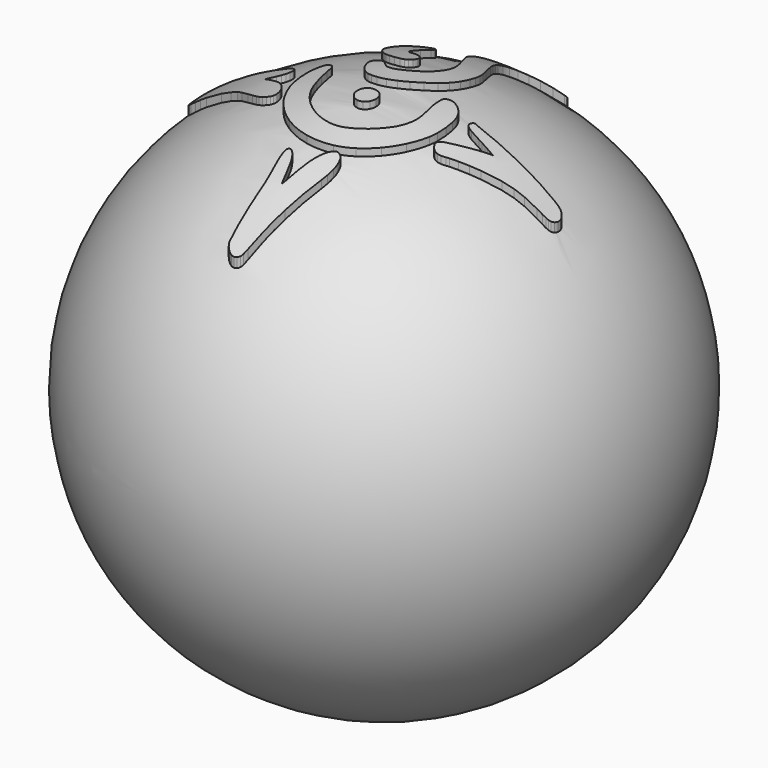
from build123d import *

# Parameters (mm, degrees)
F2_SCALE  = 33.3
F4_DEPTH  = 350
F5_SCALE  = 0.03
F8_SCALE  = 1.4
F9_R      = 2
F10_DEPTH = 25


# Not quite as in the source:
# - ends of sketch curves that miss each other by under 0.0002 mm in the source are joined


with BuildPart() as f1:
    # F0 (on Top) → F1 (revolve)
    with BuildSketch(Plane.XY):
        with BuildLine():
            ThreePointArc((0, 10), (-10, 0), (0, -10))
            Line((0, -10), (0, 10))
        make_face()
    revolve(axis=Axis((0, 0, 0), (0, 1, 0)))


with BuildPart() as f1_1:
    # F2: moved
    add(f1.part.scale(F2_SCALE))

    # F3 (on Top) → F4 (join)
    with BuildSketch(Plane.XY):
        with BuildLine():
            ThreePointArc((33.5839702777, 236.8920416086), (31.2872507857, 235.2369513176), (29.0148242928, 233.5486616119))
            ThreePointArc((29.0148242928, 233.5486616119), (19.1324774159, 225.5301798366), (9.8423522984, 216.8324557031))
            ThreePointArc((9.8423522984, 216.8324557031), (3.1177638553, 209.1003358187), (-2.5120081676, 200.5381260948))
            ThreePointArc((-2.5120081676, 200.5381260948), (-6.4438012248, 192.1284567153), (-9.0353042057, 183.2141060429))
            ThreePointArc((-9.0353042057, 183.2141060429), (-10.4367358481, 173.4113964374), (-10.5813057929, 163.510071961))
            ThreePointArc((-10.5813057929, 163.510071961), (-10.1042819519, 157.7480415442), (-9.2425675321, 152.0308749015))
            ThreePointArc((-9.2425675321, 152.0308749015), (-8.0683662262, 147.037659018), (-6.4222668913, 142.1795410427))
            ThreePointArc((-6.4222668913, 142.1795410427), (-3.8341311453, 136.1498141232), (-0.8786748343, 130.2913730901))
            ThreePointArc((-0.8786748343, 130.2913730901), (4.6685538921, 120.2474903682), (10.345759186, 110.2764991075))
            ThreePointArc((10.345759186, 110.2764991075), (14.4968308965, 102.4949690889), (18.1089318686, 94.4490799463))
            ThreePointArc((18.1089318686, 94.4490799463), (20.3325947861, 87.7758088217), (21.6547046101, 80.8671729519))
            ThreePointArc((21.6547046101, 80.8671729519), (21.933442257, 74.6170651853), (21.2348180753, 68.3998739855))
            ThreePointArc((21.2348180753, 68.3998739855), (19.5614167399, 62.0700272125), (17.0413966753, 56.0271196625))
            ThreePointArc((17.0413966753, 56.0271196625), (14.2722480259, 51.3438477785), (10.8718007094, 47.0967102684))
            ThreePointArc((10.8718007094, 47.0967102684), (6.4493698335, 42.7450902566), (1.6320588081, 38.835102261))
            ThreePointArc((1.6320588081, 38.835102261), (-3.2693678081, 35.5880451103), (-8.4647199209, 32.8356498312))
            ThreePointArc((-8.4647199209, 32.8356498312), (-12.6861471562, 31.3957563266), (-17.119585, 30.9075252801))
            ThreePointArc((-17.119585, 30.9075252801), (-18.5749981899, 30.9588179082), (-20.0231380929, 31.1129263476))
            ThreePointArc((-20.0231380929, 31.1129263476), (-21.0800039659, 31.3548811444), (-22.081829036, 31.7694339301))
            ThreePointArc((-22.081829036, 31.7694339301), (-23.2085403851, 32.4340347627), (-24.2524288095, 33.2223682244))
            ThreePointArc((-24.2524288095, 33.2223682244), (-26.1201182917, 34.8396411796), (-27.9553924433, 36.4936075178))
            ThreePointArc((-27.9553924433, 36.4936075178), (-29.6511377796, 38.0243808047), (-31.3744037529, 39.5241052892))
            ThreePointArc((-31.3744037529, 39.5241052892), (-32.3603682601, 40.2870956891), (-33.4155611268, 40.9510597751))
            ThreePointArc((-33.4155611268, 40.9510597751), (-34.1958978055, 41.3006066899), (-35.0270239713, 41.5014491964))
            ThreePointArc((-35.0270239713, 41.5014491964), (-35.8658550267, 41.5417572719), (-36.6967041013, 41.4194784081))
            ThreePointArc((-36.6967041013, 41.4194784081), (-37.9964275162, 40.9976995728), (-39.2238602532, 40.3972104365))
            ThreePointArc((-39.2238602532, 40.3972104365), (-40.4233299971, 39.6010223307), (-41.5180846961, 38.6660596848))
            ThreePointArc((-41.5180846961, 38.6660596848), (-42.4537917331, 37.6433007258), (-43.2545310552, 36.5117530341))
            ThreePointArc((-43.2545310552, 36.5117530341), (-43.7991045433, 35.4185857778), (-44.1365958304, 34.2448419676))
            ThreePointArc((-44.1365958304, 34.2448419676), (-44.3311387679, 31.90950028), (-44.0309948562, 29.5853700343))
            ThreePointArc((-44.0309948562, 29.5853700343), (-43.1598026618, 26.5326639584), (-42.0249300746, 23.5678614015))
            ThreePointArc((-42.0249300746, 23.5678614015), (-40.4982189899, 20.4151830954), (-38.7147278348, 17.4003221072))
            ThreePointArc((-38.7147278348, 17.4003221072), (-36.7627376663, 14.6873048367), (-34.5602718697, 12.1733691257))
            ThreePointArc((-34.5602718697, 12.1733691257), (-32.4972285983, 10.2580065105), (-30.2358389338, 8.5814391004))
            ThreePointArc((-30.2358389338, 8.5814391004), (-27.9386033944, 7.2780681906), (-25.4883721848, 6.2919474347))
            ThreePointArc((-25.4883721848, 6.2919474347), (-22.7235404396, 5.5680825845), (-19.8920639941, 5.179475077))
            ThreePointArc((-19.8920639941, 5.179475077), (-16.4407701729, 5.0330128077), (-12.9875269897, 5.1224098294))
            ThreePointArc((-12.9875269897, 5.1224098294), (-7.7263055039, 5.755509923), (-2.5780300379, 7.0111081229))
            ThreePointArc((-2.5780300379, 7.0111081229), (2.7682669976, 8.9466005626), (7.9024667665, 11.389757435))
            ThreePointArc((7.9024667665, 11.389757435), (13.2958214566, 14.5927578538), (18.3915086938, 18.2508253897))
            ThreePointArc((18.3915086938, 18.2508253897), (23.754147094, 22.7429501279), (28.8251250537, 27.5618979469))
            ThreePointArc((28.8251250537, 27.5618979469), (33.4797468923, 32.7068050735), (37.6624816046, 38.2421735837))
            ThreePointArc((37.6624816046, 38.2421735837), (41.0387740077, 43.7658663194), (43.7964406901, 49.6229821258))
            ThreePointArc((43.7964406901, 49.6229821258), (45.904591086, 55.7482763417), (47.336918584, 62.0658680708))
            ThreePointArc((47.336918584, 62.0658680708), (48.2013923808, 68.9616610524), (48.4567558849, 75.9067360064))
            ThreePointArc((48.4567558849, 75.9067360064), (48.2830243872, 80.8780020701), (47.8342436997, 85.832017083))
            ThreePointArc((47.8342436997, 85.832017083), (47.1370175393, 90.2919899618), (46.1117340455, 94.6881560124))
            ThreePointArc((46.1117340455, 94.6881560124), (44.6916033909, 99.2773499841), (42.963369873, 103.759612946))
            ThreePointArc((42.963369873, 103.759612946), (40.5613501018, 109.1298002215), (37.9608576069, 114.4067357971))
            ThreePointArc((37.9608576069, 114.4067357971), (32.6470866927, 124.7414153072), (27.3662677803, 135.0929713965))
            ThreePointArc((27.3662677803, 135.0929713965), (24.7259502515, 140.4197225176), (22.1922672104, 145.7980126376))
            ThreePointArc((22.1922672104, 145.7980126376), (20.6601677307, 149.3164912102), (19.2672299611, 152.8923469857))
            ThreePointArc((19.2672299611, 152.8923469857), (18.2940235081, 155.868538738), (17.536259209, 158.9067358325))
            ThreePointArc((17.536259209, 158.9067358325), (16.7190998594, 163.8904603666), (16.3642416365, 168.9282510154))
            ThreePointArc((16.3642416365, 168.9282510154), (16.5213414737, 173.607931726), (17.2169992309, 178.2382829515))
            ThreePointArc((17.2169992309, 178.2382829515), (18.4910489703, 183.0168650293), (20.2695342301, 187.6315198968))
            ThreePointArc((20.2695342301, 187.6315198968), (22.8296254351, 192.8726243488), (25.7284907636, 197.9342271459))
            ThreePointArc((25.7284907636, 197.9342271459), (28.9537669376, 203.2502120973), (32.0973782481, 208.6148938572))
            ThreePointArc((32.0973782481, 208.6148938572), (35.3789821615, 214.3978703308), (38.5879989981, 220.221439001))
            ThreePointArc((38.5879989981, 220.221439001), (41.5839102506, 225.7709084772), (44.5535395691, 231.3344862287))
            ThreePointArc((44.5535395691, 231.3344862287), (44.9905118903, 232.4747939041), (45.139103, 233.686886))
            ThreePointArc((45.139103, 233.686886), (45.0470188997, 234.6434926782), (44.774146878, 235.5649679507))
            ThreePointArc((44.774146878, 235.5649679507), (44.3211975486, 236.4606147714), (43.7242942718, 237.267493239))
            ThreePointArc((43.7242942718, 237.267493239), (42.9700203597, 237.9983716709), (42.1090869519, 238.5999579178))
            ThreePointArc((42.1090869519, 238.5999579178), (41.1398732263, 239.0758936063), (40.1113668985, 239.4046255777))
            ThreePointArc((40.1113668985, 239.4046255777), (39.2636176129, 239.5027838805), (38.4169479014, 239.3957113921))
            ThreePointArc((38.4169479014, 239.3957113921), (37.3828331438, 239.0688465307), (36.3951172895, 238.6209054515))
            ThreePointArc((36.3951172895, 238.6209054515), (34.9610957305, 237.8027303056), (33.5839702777, 236.8920416086))
        make_face()
        with BuildLine():
            ThreePointArc((-42.323086763, 129.1738635543), (-44.1393310136, 128.1627035744), (-45.9151157273, 127.0820665709))
            ThreePointArc((-45.9151157273, 127.0820665709), (-50.1260663332, 123.9751883225), (-53.8649160591, 120.3137950525))
            ThreePointArc((-53.8649160591, 120.3137950525), (-57.1547961085, 116.086062654), (-59.8694062449, 111.4678461233))
            ThreePointArc((-59.8694062449, 111.4678461233), (-62.0590099734, 106.3507303256), (-63.5973965422, 101.0016551201))
            ThreePointArc((-63.5973965422, 101.0016551201), (-64.540269546, 95.2728172325), (-64.8511271886, 89.475235001))
            ThreePointArc((-64.8511271886, 89.475235001), (-64.7217148896, 86.1283645355), (-64.3423022831, 82.800552109))
            ThreePointArc((-64.3423022831, 82.800552109), (-63.7415741406, 79.9469143788), (-62.8227642257, 77.1792599106))
            ThreePointArc((-62.8227642257, 77.1792599106), (-61.6381479464, 74.6412940159), (-60.1599131773, 72.2623428746))
            ThreePointArc((-60.1599131773, 72.2623428746), (-58.3046440662, 69.8898008927), (-56.2304288842, 67.7060861211))
            ThreePointArc((-56.2304288842, 67.7060861211), (-54.0105104417, 65.773116141), (-51.6200521128, 64.0555248264))
            ThreePointArc((-51.6200521128, 64.0555248264), (-49.1742690519, 62.6436953185), (-46.5932000138, 61.4977459638))
            ThreePointArc((-46.5932000138, 61.4977459638), (-43.7334124454, 60.5616789062), (-40.7961929219, 59.9079604538))
            ThreePointArc((-40.7961929219, 59.9079604538), (-37.3402905378, 59.4244636968), (-33.8608970037, 59.1582849169))
            ThreePointArc((-33.8608970037, 59.1582849169), (-30.4947947909, 59.1071918916), (-27.1316409481, 59.2570283034))
            ThreePointArc((-27.1316409481, 59.2570283034), (-24.751118399, 59.6244431369), (-22.4577052097, 60.3607425109))
            ThreePointArc((-22.4577052097, 60.3607425109), (-20.6603123938, 61.3237138367), (-19.0963994382, 62.6321904263))
            ThreePointArc((-19.0963994382, 62.6321904263), (-17.6609824972, 64.3557127269), (-16.5077638595, 66.2795209299))
            ThreePointArc((-16.5077638595, 66.2795209299), (-15.3983275477, 69.5915453697), (-15.244384476, 73.0810520502))
            ThreePointArc((-15.244384476, 73.0810520502), (-16.082111947, 76.3310753547), (-17.8814891709, 79.1642148493))
            ThreePointArc((-17.8814891709, 79.1642148493), (-20.7510205353, 81.6786214229), (-24.1658758241, 83.3801545075))
            ThreePointArc((-24.1658758241, 83.3801545075), (-28.476842514, 84.4896681468), (-32.9108970048, 84.8828782833))
            ThreePointArc((-32.9108970048, 84.8828782833), (-34.8638480241, 85.0972267848), (-36.7321522372, 85.7050114648))
            ThreePointArc((-36.7321522372, 85.7050114648), (-37.8925119396, 86.5936733865), (-38.520753509, 87.9133198927))
            ThreePointArc((-38.520753509, 87.9133198927), (-38.8051473858, 90.2299034154), (-38.6901994324, 92.5610460587))
            ThreePointArc((-38.6901994324, 92.5610460587), (-37.8645814012, 98.300986598), (-36.9486449169, 104.027208986))
            ThreePointArc((-36.9486449169, 104.027208986), (-35.782735233, 111.040672784), (-34.6414639317, 118.058187989))
            ThreePointArc((-34.6414639317, 118.058187989), (-34.3563734984, 120.2908381466), (-34.216723267, 122.5372800079))
            ThreePointArc((-34.216723267, 122.5372800079), (-34.3215228193, 123.8518411353), (-34.7086034039, 125.1124848258))
            ThreePointArc((-34.7086034039, 125.1124848258), (-35.3742530506, 126.3261369302), (-36.2562315231, 127.3929804769))
            ThreePointArc((-36.2562315231, 127.3929804769), (-37.3148410074, 128.3560169381), (-38.459579028, 129.2148929587))
            ThreePointArc((-38.459579028, 129.2148929587), (-39.3071587518, 129.6131794979), (-40.2363500056, 129.729915175))
            ThreePointArc((-40.2363500056, 129.729915175), (-41.311585159, 129.5714780139), (-42.323086763, 129.1738635543))
        make_face()
        with BuildLine():
            ThreePointArc((71.5374891, 21.784049359), (68.4658131544, 22.1052264829), (65.4591599138, 21.399263205))
            ThreePointArc((65.4591599138, 21.399263205), (64.8462780768, 21.1153380792), (64.2552783109, 20.7882954827))
            ThreePointArc((64.2552783109, 20.7882954827), (63.681590073, 20.4159346469), (63.1349283205, 20.004921603))
            ThreePointArc((63.1349283205, 20.004921603), (62.6763267243, 19.6062086451), (62.2480107529, 19.1751252283))
            ThreePointArc((62.2480107529, 19.1751252283), (61.983246262, 18.8274765548), (61.7887640545, 18.4361499791))
            ThreePointArc((61.7887640545, 18.4361499791), (61.2868613687, 16.6681879497), (61.1088458097, 14.8390060014))
            ThreePointArc((61.1088458097, 14.8390060014), (61.1467310964, 11.6318619774), (61.3066211357, 8.4284820094))
            ThreePointArc((61.3066211357, 8.4284820094), (61.6502355818, 4.5030127094), (62.1381356951, 0.5928549562))
            ThreePointArc((62.1381356951, 0.5928549562), (62.8215632419, -3.7599736308), (63.6195513604, -8.0932639287))
            ThreePointArc((63.6195513604, -8.0932639287), (64.5281963728, -12.9898389402), (65.3208385892, -17.9065249121))
            ThreePointArc((65.3208385892, -17.9065249121), (65.7590382663, -21.5591230569), (65.9875589573, -25.2308080014))
            ThreePointArc((65.9875589573, -25.2308080014), (65.9787753789, -28.3308949914), (65.7447022245, -31.4221449128))
            ThreePointArc((65.7447022245, -31.4221449128), (65.2858081574, -34.5072356367), (64.6079105693, -37.5517098878))
            ThreePointArc((64.6079105693, -37.5517098878), (61.01399806, -47.2558707002), (55.5659069706, -56.0538959775))
            ThreePointArc((55.5659069706, -56.0538959775), (47.8299635042, -64.8004670149), (38.9517282463, -72.3849423327))
            ThreePointArc((38.9517282463, -72.3849423327), (29.2915650966, -78.5229773809), (18.8590259121, -83.2300307612))
            ThreePointArc((18.8590259121, -83.2300307612), (9.3869186219, -85.5342358468), (-0.3608969228, -85.6355692582))
            ThreePointArc((-0.3608969228, -85.6355692582), (-9.010903134, -84.1236834026), (-17.3690077824, -81.4310094568))
            ThreePointArc((-17.3690077824, -81.4310094568), (-25.6033621568, -77.5241805181), (-33.2910371528, -72.62851321))
            ThreePointArc((-33.2910371528, -72.62851321), (-40.3490129192, -66.7938709816), (-46.6349295908, -60.1346424924))
            ThreePointArc((-46.6349295908, -60.1346424924), (-51.8605469173, -52.9316919318), (-56.0734585258, -45.0932642386))
            ThreePointArc((-56.0734585258, -45.0932642386), (-57.4451497455, -41.8533716584), (-58.6502294459, -38.5478878138))
            ThreePointArc((-58.6502294459, -38.5478878138), (-59.975765752, -34.4163318357), (-61.1877121377, -30.250040038))
            ThreePointArc((-61.1877121377, -30.250040038), (-62.5131053839, -25.2245803402), (-63.7222743719, -20.1698970844))
            ThreePointArc((-63.7222743719, -20.1698970844), (-65.047563345, -14.1404547802), (-66.2893554165, -8.0932638844))
            ThreePointArc((-66.2893554165, -8.0932638844), (-67.2129145298, -3.7222824225), (-68.246389156, 0.6240229608))
            ThreePointArc((-68.246389156, 0.6240229608), (-68.9862952936, 2.8656925532), (-70.0434155326, 4.9763892783))
            ThreePointArc((-70.0434155326, 4.9763892783), (-71.0608013707, 6.225445276), (-72.395516058, 7.1275268794))
            ThreePointArc((-72.395516058, 7.1275268794), (-74.0622973305, 7.7094701823), (-75.816693, 7.906736))
            ThreePointArc((-75.816693, 7.906736), (-77.163837917, 7.7442241254), (-78.4336889578, 7.266010919))
            ThreePointArc((-78.4336889578, 7.266010919), (-79.5410932031, 6.5027734199), (-80.4288245577, 5.4924226989))
            ThreePointArc((-80.4288245577, 5.4924226989), (-81.3962666094, 3.8387328595), (-82.1294209382, 2.0686709792))
            ThreePointArc((-82.1294209382, 2.0686709792), (-83.1063236606, -0.9975207464), (-83.9850977593, -4.0932640642))
            ThreePointArc((-83.9850977593, -4.0932640642), (-85.0973792104, -9.0140758592), (-85.8291828043, -14.0056710211))
            ThreePointArc((-85.8291828043, -14.0056710211), (-86.250156855, -19.4579352569), (-86.3418168172, -24.9256589976))
            ThreePointArc((-86.3418168172, -24.9256589976), (-86.1040704543, -30.3773359601), (-85.5377104276, -35.8047240577))
            ThreePointArc((-85.5377104276, -35.8047240577), (-84.6745063003, -40.7400982364), (-83.4295883128, -45.5932640934))
            ThreePointArc((-83.4295883128, -45.5932640934), (-77.1275119295, -61.1364788468), (-67.9999647766, -75.2075688228))
            ThreePointArc((-67.9999647766, -75.2075688228), (-56.2237578571, -87.5815805814), (-42.4207551489, -97.6449962484))
            ThreePointArc((-42.4207551489, -97.6449962484), (-27.0523645676, -105.0629018059), (-10.6024598518, -109.6030981815))
            ThreePointArc((-10.6024598518, -109.6030981815), (6.0699693912, -110.9975263888), (22.7033590197, -109.1962270955))
            ThreePointArc((22.7033590197, -109.1962270955), (34.1805002574, -105.8709169672), (44.9967483061, -100.7924095378))
            ThreePointArc((44.9967483061, -100.7924095378), (55.5307329402, -93.8299830206), (65.0470770701, -85.5306210703))
            ThreePointArc((65.0470770701, -85.5306210703), (73.6088336423, -75.8126204442), (80.8430690572, -65.0697600333))
            ThreePointArc((80.8430690572, -65.0697600333), (86.5475762627, -53.5872552171), (90.6723633348, -41.4474260893))
            ThreePointArc((90.6723633348, -41.4474260893), (91.8745230209, -36.0089566229), (92.6027769596, -30.4870199964))
            ThreePointArc((92.6027769596, -30.4870199964), (92.9606828713, -24.2463071513), (92.935869588, -17.9953889796))
            ThreePointArc((92.935869588, -17.9953889796), (92.5338365455, -11.8695224861), (91.7537819012, -5.7802380158))
            ThreePointArc((91.7537819012, -5.7802380158), (90.6732899547, -0.6674106462), (89.0885668329, 4.3122599375))
            ThreePointArc((89.0885668329, 4.3122599375), (87.2023114541, 8.43517302), (84.7511321201, 12.2493690898))
            ThreePointArc((84.7511321201, 12.2493690898), (81.8304414076, 15.5938280832), (78.4392089762, 18.4600769671))
            ThreePointArc((78.4392089762, 18.4600769671), (75.1360266216, 20.4286930308), (71.5374891, 21.784049359))
        make_face()
        with BuildLine():
            ThreePointArc((104.8142318479, 11.9091901033), (104.3045345563, 11.1064301641), (103.8456058546, 10.2736040743))
            ThreePointArc((103.8456058546, 10.2736040743), (103.1951350823, 8.1752489911), (103.29054642, 5.9804590919))
            ThreePointArc((103.29054642, 5.9804590919), (104.1267322308, 4.0221396846), (105.6238820501, 2.5079520727))
            ThreePointArc((105.6238820501, 2.5079520727), (108.5772374837, 0.8209525428), (111.7710488812, -0.3485964341))
            ThreePointArc((111.7710488812, -0.3485964341), (117.4304015267, -1.7846574056), (123.1391030031, -3.009920984))
            ThreePointArc((123.1391030031, -3.009920984), (125.3435930294, -3.4416528583), (127.5476389708, -3.8756461479))
            ThreePointArc((127.5476389708, -3.8756461479), (129.8295442062, -4.3272815369), (132.1110310637, -4.7810256807))
            ThreePointArc((132.1110310637, -4.7810256807), (134.1562517695, -5.1897456832), (136.201093094, -5.6003595329))
            ThreePointArc((136.201093094, -5.6003595329), (137.5695339019, -5.8778954343), (138.9371558755, -6.1594386005))
            Line((138.9371558755, -6.1594386005), (144.235209, -7.258204))
            Line((144.235209, -7.258204), (138.591474, -11.211653))
            ThreePointArc((138.591474, -11.211653), (137.1751082294, -12.2125774263), (135.7670702137, -13.2251832946))
            ThreePointArc((135.7670702137, -13.2251832946), (133.7661933934, -14.6812406359), (131.7696298116, -16.1432067435))
            ThreePointArc((131.7696298116, -16.1432067435), (129.5841404587, -17.7534143292), (127.4033812145, -19.3700222885))
            ThreePointArc((127.4033812145, -19.3700222885), (125.345734985, -20.9055864378), (123.2934207479, -22.4482696658))
            ThreePointArc((123.2934207479, -22.4482696658), (121.2249623102, -23.9997790182), (119.1479861361, -25.5398671847))
            ThreePointArc((119.1479861361, -25.5398671847), (116.9147547854, -27.1785866436), (114.6741980184, -28.8072760254))
            ThreePointArc((114.6741980184, -28.8072760254), (112.603473458, -30.2982972258), (110.5260159372, -31.7799229115))
            ThreePointArc((110.5260159372, -31.7799229115), (109.0234332538, -32.8331367522), (107.5085110291, -33.8685230431))
            ThreePointArc((107.5085110291, -33.8685230431), (104.9108803997, -35.8133566578), (102.5161541179, -38.0031851169))
            ThreePointArc((102.5161541179, -38.0031851169), (101.1805879935, -39.800294476), (100.4016803976, -41.8994948695))
            ThreePointArc((100.4016803976, -41.8994948695), (100.3060734578, -43.9436416723), (100.884527141, -45.9065649313))
            ThreePointArc((100.884527141, -45.9065649313), (102.2452566737, -48.2393711896), (103.9385390836, -50.3432639217))
            ThreePointArc((103.9385390836, -50.3432639217), (105.2921971148, -51.5289299385), (106.852567356, -52.425277208))
            ThreePointArc((106.852567356, -52.425277208), (108.5001219929, -52.955592022), (110.2240250012, -53.109958053))
            ThreePointArc((110.2240250012, -53.109958053), (112.2079708743, -52.8873074636), (114.1199851153, -52.3130112871))
            ThreePointArc((114.1199851153, -52.3130112871), (116.4055431731, -51.2713103284), (118.5861261387, -50.0247252187))
            ThreePointArc((118.5861261387, -50.0247252187), (120.1522837174, -49.0751986092), (121.7554278239, -48.1895466655))
            ThreePointArc((121.7554278239, -48.1895466655), (125.8186540708, -46.0599419228), (129.8895797923, -43.9450925984))
            ThreePointArc((129.8895797923, -43.9450925984), (134.7571909927, -41.4420836404), (139.6365420311, -38.9620380616))
            ThreePointArc((139.6365420311, -38.9620380616), (144.9490585908, -36.2898059807), (150.2713621894, -33.6371203818))
            ThreePointArc((150.2713621894, -33.6371203818), (159.771973215, -28.9932028933), (169.3266017599, -24.4614644861))
            ThreePointArc((169.3266017599, -24.4614644861), (175.2071418209, -21.8851639761), (181.2048411237, -19.5948193488))
            ThreePointArc((181.2048411237, -19.5948193488), (186.4762014226, -17.911544417), (191.8434050268, -16.5647781231))
            ThreePointArc((191.8434050268, -16.5647781231), (198.6725640104, -15.1933026657), (205.5421930927, -14.0415416133))
            ThreePointArc((205.5421930927, -14.0415416133), (208.7890078017, -13.5303673435), (212.0293680137, -12.9797580775))
            ThreePointArc((212.0293680137, -12.9797580775), (213.8742350037, -12.5997124067), (215.6941988997, -12.1142226632))
            ThreePointArc((215.6941988997, -12.1142226632), (216.9170994822, -11.6810062953), (218.0895260506, -11.1255080941))
            ThreePointArc((218.0895260506, -11.1255080941), (219.0600236711, -10.5082898568), (219.9304314898, -9.7564824898))
            ThreePointArc((219.9304314898, -9.7564824898), (221.1130817951, -8.2960700231), (221.9662960027, -6.6217070011))
            ThreePointArc((221.9662960027, -6.6217070011), (222.5938484988, -4.5656080347), (222.926912449, -2.4418299529))
            ThreePointArc((222.926912449, -2.4418299529), (222.9622194782, -0.2513031537), (222.6953960959, 1.9231990186))
            ThreePointArc((222.6953960959, 1.9231990186), (222.1395047052, 3.8301496826), (221.2425109841, 5.60240199))
            ThreePointArc((221.2425109841, 5.60240199), (219.7273027314, 7.6494400847), (217.9188649594, 9.4426979523))
            ThreePointArc((217.9188649594, 9.4426979523), (216.1284414843, 10.608931275), (214.1015529638, 11.2852738163))
            ThreePointArc((214.1015529638, 11.2852738163), (210.8598093354, 11.760952764), (207.5871610002, 11.918892571))
            ThreePointArc((207.5871610002, 11.918892571), (198.7326844289, 11.8815327774), (189.8787279915, 11.778544551))
            ThreePointArc((189.8787279915, 11.778544551), (175.6317937987, 11.5923787772), (161.3841609978, 11.47092436))
            ThreePointArc((161.3841609978, 11.47092436), (148.64321383, 11.4316662809), (135.9022739971, 11.4732375555))
            ThreePointArc((135.9022739971, 11.4732375555), (125.0130277709, 11.5605324865), (114.1241120016, 11.6822581226))
            ThreePointArc((114.1241120016, 11.6822581226), (111.5332283864, 11.8535026633), (108.9752179916, 12.2991319634))
            ThreePointArc((108.9752179916, 12.2991319634), (107.8797024364, 12.5266579985), (106.7756219312, 12.7081205188))
            ThreePointArc((106.7756219312, 12.7081205188), (106.2023348357, 12.7152584806), (105.6463432226, 12.5753214362))
            ThreePointArc((105.6463432226, 12.5753214362), (105.1801211305, 12.30492226), (104.8142318479, 11.9091901033))
        make_face()
        with BuildLine():
            ThreePointArc((-117.9514469773, -5.0865513471), (-124.6760136988, -5.6988847953), (-131.3608969489, -6.6512953035))
            ThreePointArc((-131.3608969489, -6.6512953035), (-133.5908593712, -6.9929873982), (-135.8299740043, -7.2683989603))
            ThreePointArc((-135.8299740043, -7.2683989603), (-139.7238664088, -7.6763270622), (-143.6202720786, -8.0595061741))
            ThreePointArc((-143.6202720786, -8.0595061741), (-148.1388614269, -8.4742718919), (-152.6601029727, -8.8590513341))
            ThreePointArc((-152.6601029727, -8.8590513341), (-157.2594050256, -9.22051267), (-161.8608969782, -9.5529363149))
            ThreePointArc((-161.8608969782, -9.5529363149), (-173.2089697642, -10.3684065831), (-184.5523419628, -11.2468454639))
            ThreePointArc((-184.5523419628, -11.2468454639), (-192.6881107586, -11.9591968665), (-200.8126559317, -12.7898256237))
            ThreePointArc((-200.8126559317, -12.7898256237), (-206.716176635, -13.4765624294), (-212.6100450074, -14.2417289455))
            ThreePointArc((-212.6100450074, -14.2417289455), (-214.7770267055, -14.7288696558), (-216.8297198203, -15.5771423476))
            ThreePointArc((-216.8297198203, -15.5771423476), (-219.4760480652, -17.5318650988), (-221.3787825206, -20.2158167435))
            ThreePointArc((-221.3787825206, -20.2158167435), (-222.5977853264, -23.6570502339), (-222.9834616629, -27.2873819961))
            ThreePointArc((-222.9834616629, -27.2873819961), (-222.5135604511, -30.8748168794), (-221.2126042669, -34.2509106122))
            ThreePointArc((-221.2126042669, -34.2509106122), (-219.2528164445, -36.8191112291), (-216.5657068922, -38.6123947607))
            ThreePointArc((-216.5657068922, -38.6123947607), (-215.4785081926, -39.0334157708), (-214.3523961301, -39.3352956158))
            ThreePointArc((-214.3523961301, -39.3352956158), (-211.025018147, -40.0259918243), (-207.6929350273, -40.6936201387))
            ThreePointArc((-207.6929350273, -40.6936201387), (-203.7065777428, -41.4571772051), (-199.712741004, -42.1805940226))
            ThreePointArc((-199.712741004, -42.1805940226), (-195.2895926024, -42.9418456244), (-190.8608970789, -43.6701324913))
            ThreePointArc((-190.8608970789, -43.6701324913), (-179.9789572818, -45.4557835588), (-169.1093370338, -47.3149551938))
            ThreePointArc((-169.1093370338, -47.3149551938), (-161.8816855346, -48.6571153847), (-154.6847820623, -50.155421284))
            ThreePointArc((-154.6847820623, -50.155421284), (-149.4479180908, -51.3934012257), (-144.253500079, -52.7988762745))
            ThreePointArc((-144.253500079, -52.7988762745), (-140.0777860257, -54.1352872598), (-135.9879521301, -55.7151103094))
            ThreePointArc((-135.9879521301, -55.7151103094), (-130.4693096471, -58.0091789989), (-124.9320371405, -60.2579073501))
            ThreePointArc((-124.9320371405, -60.2579073501), (-120.7145643577, -61.9053945924), (-116.4673249543, -63.4745498727))
            ThreePointArc((-116.4673249543, -63.4745498727), (-113.2483723023, -64.5880257571), (-110.0044211462, -65.6264214756))
            ThreePointArc((-110.0044211462, -65.6264214756), (-107.8265027735, -66.2063775677), (-105.6108968846, -66.6196182175))
            ThreePointArc((-105.6108968846, -66.6196182175), (-103.2513744781, -66.876592022), (-100.8791539974, -66.9537394768))
            ThreePointArc((-100.8791539974, -66.9537394768), (-98.5353380571, -66.848663632), (-96.2070230571, -66.5597636522))
            ThreePointArc((-96.2070230571, -66.5597636522), (-94.2041502525, -66.1427594092), (-92.2439048396, -65.5572424642))
            ThreePointArc((-92.2439048396, -65.5572424642), (-90.9290764338, -64.9287176437), (-89.7888150121, -64.0211819879))
            ThreePointArc((-89.7888150121, -64.0211819879), (-88.5541332889, -62.2550233694), (-88.0011321234, -60.1722499896))
            ThreePointArc((-88.0011321234, -60.1722499896), (-88.0220059027, -57.4796714432), (-88.5350956665, -54.8363489028))
            ThreePointArc((-88.5350956665, -54.8363489028), (-89.6618472568, -51.8337503096), (-91.2262640747, -49.0341490494))
            ThreePointArc((-91.2262640747, -49.0341490494), (-93.2803841357, -46.3203976304), (-95.659537253, -43.8865762806))
            ThreePointArc((-95.659537253, -43.8865762806), (-97.7229136894, -42.1466932872), (-99.8970354334, -40.5473466321))
            ThreePointArc((-99.8970354334, -40.5473466321), (-102.1475888147, -39.1150990405), (-104.4911121144, -37.8406492287))
            ThreePointArc((-104.4911121144, -37.8406492287), (-107.3393460315, -36.5120947348), (-110.2558439232, -35.3409697926))
            ThreePointArc((-110.2558439232, -35.3409697926), (-114.23633615, -33.919211312), (-118.2484319164, -32.5892477376))
            Line((-118.2484319164, -32.5892477376), (-128.135967, -29.437193))
            Line((-128.135967, -29.437193), (-122.475024, -27.139585))
            ThreePointArc((-122.475024, -27.139585), (-119.7764581095, -25.9590433218), (-117.1450900435, -24.6354729191))
            ThreePointArc((-117.1450900435, -24.6354729191), (-114.9303210407, -23.3286487567), (-112.8276630125, -21.8481689836))
            ThreePointArc((-112.8276630125, -21.8481689836), (-111.1284174541, -20.4151569797), (-109.5709641968, -18.8291878241))
            ThreePointArc((-109.5709641968, -18.8291878241), (-108.3920188786, -17.303254781), (-107.4428498798, -15.6247250571))
            ThreePointArc((-107.4428498798, -15.6247250571), (-106.6454089976, -12.8331857693), (-106.7944858369, -9.9338101838))
            ThreePointArc((-106.7944858369, -9.9338101838), (-107.9175848315, -7.6957769904), (-109.9730897689, -6.2657263841))
            ThreePointArc((-109.9730897689, -6.2657263841), (-113.8994808466, -5.2513150263), (-117.9514469773, -5.0865513471))
        make_face()
        with BuildLine():
            ThreePointArc((-2.0594129272, -17.4331663857), (-4.5563011175, -18.2463611906), (-6.7652848125, -19.6662652229))
            ThreePointArc((-6.7652848125, -19.6662652229), (-9.2030586476, -22.3991412941), (-10.7714662054, -25.7084389365))
            ThreePointArc((-10.7714662054, -25.7084389365), (-11.3477223282, -29.3329206964), (-10.8852468991, -32.9736699723))
            ThreePointArc((-10.8852468991, -32.9736699723), (-9.4155015807, -36.3666541314), (-7.0629733312, -39.2193903621))
            ThreePointArc((-7.0629733312, -39.2193903621), (-4.0034964573, -41.3212757926), (-0.4850458843, -42.5039953832))
            ThreePointArc((-0.4850458843, -42.5039953832), (2.9852948545, -42.6225473), (6.3332929937, -41.7015539858))
            ThreePointArc((6.3332929937, -41.7015539858), (9.3715370055, -39.8052817997), (11.7768116924, -37.1517127904))
            ThreePointArc((11.7768116924, -37.1517127904), (13.4274451136, -33.8639407263), (14.1569222654, -30.2581260177))
            ThreePointArc((14.1569222654, -30.2581260177), (13.9044682796, -26.6174442381), (12.6831537319, -23.1784491386))
            ThreePointArc((12.6831537319, -23.1784491386), (11.2124415942, -21.0898009607), (9.2338468708, -19.4740632115))
            ThreePointArc((9.2338468708, -19.4740632115), (6.6170985816, -18.1903942511), (3.8089259633, -17.4097892033))
            ThreePointArc((3.8089259633, -17.4097892033), (0.8736860788, -17.1527711741), (-2.0594129272, -17.4331663857))
        make_face()
        with BuildLine():
            ThreePointArc((30.1499251378, -114.6352613144), (28.796184359, -115.2836076283), (27.4890931586, -116.0214962601))
            ThreePointArc((27.4890931586, -116.0214962601), (24.9394888607, -117.915194701), (22.7760160893, -120.240267069))
            ThreePointArc((22.7760160893, -120.240267069), (20.4067273321, -123.5935872724), (18.3344272913, -127.1381406256))
            ThreePointArc((18.3344272913, -127.1381406256), (16.0841786964, -131.7755062902), (14.1566139976, -136.5560159991))
            ThreePointArc((14.1566139976, -136.5560159991), (12.0989319596, -142.5542264819), (10.2651952063, -148.6246460582))
            ThreePointArc((10.2651952063, -148.6246460582), (8.7030279125, -154.1288184746), (7.1217599039, -159.6275339722))
            ThreePointArc((7.1217599039, -159.6275339722), (6.33224659, -162.2286473842), (5.4756813209, -164.8084571112))
            ThreePointArc((5.4756813209, -164.8084571112), (5.0134523298, -165.9961179877), (4.4632103046, -167.1456516344))
            ThreePointArc((4.4632103046, -167.1456516344), (4.1474869671, -167.3179555794), (3.8666238176, -167.0932640582))
            ThreePointArc((3.8666238176, -167.0932640582), (3.7112624604, -166.5958325835), (3.5620534099, -166.0965211724))
            ThreePointArc((3.5620534099, -166.0965211724), (3.149375733, -164.6815882972), (2.7378977384, -163.2663060759))
            ThreePointArc((2.7378977384, -163.2663060759), (2.2490135308, -161.5783003149), (1.7621724528, -159.8897041574))
            ThreePointArc((1.7621724528, -159.8897041574), (1.2284051547, -158.0309469796), (0.6963289991, -156.1717050003))
            ThreePointArc((0.6963289991, -156.1717050003), (-1.1651919267, -150.2695865956), (-3.3454467528, -144.4776308992))
            ThreePointArc((-3.3454467528, -144.4776308992), (-5.4241594451, -140.0980173385), (-7.9783489213, -135.9775589449))
            ThreePointArc((-7.9783489213, -135.9775589449), (-10.1053723125, -133.4489264142), (-12.6446557103, -131.3346295818))
            ThreePointArc((-12.6446557103, -131.3346295818), (-14.7188184177, -130.6207577703), (-16.8608971018, -131.0932638098))
            ThreePointArc((-16.8608971018, -131.0932638098), (-17.8825744707, -131.9718562803), (-18.4355492036, -133.2006639579))
            ThreePointArc((-18.4355492036, -133.2006639579), (-18.7498699533, -135.3437940606), (-18.8123505126, -137.5089499856))
            ThreePointArc((-18.8123505126, -137.5089499856), (-18.595417036, -140.9316488936), (-18.148071248, -144.3319150412))
            ThreePointArc((-18.148071248, -144.3319150412), (-17.1960739094, -149.7691438734), (-16.1489153965, -155.1888500802))
            ThreePointArc((-16.1489153965, -155.1888500802), (-15.3140631148, -159.574207185), (-14.5803259659, -163.9776109947))
            ThreePointArc((-14.5803259659, -163.9776109947), (-14.1181667143, -167.4895260381), (-13.8163225027, -171.0188359689))
            ThreePointArc((-13.8163225027, -171.0188359689), (-13.5932048142, -175.5618880745), (-13.4926446533, -180.109303997))
            ThreePointArc((-13.4926446533, -180.109303997), (-13.4282672751, -189.601197534), (-13.3989149774, -199.093264))
            ThreePointArc((-13.3989149774, -199.093264), (-13.3745060449, -206.1306000392), (-13.3188092467, -213.1677580025))
            ThreePointArc((-13.3188092467, -213.1677580025), (-13.2380294736, -217.9756396663), (-13.093189568, -222.7820180209))
            ThreePointArc((-13.093189568, -222.7820180209), (-12.9479881823, -226.2458988347), (-12.7674362756, -229.7081170158))
            ThreePointArc((-12.7674362756, -229.7081170158), (-12.5957922056, -230.6838563429), (-12.2027190655, -231.5932640379))
            ThreePointArc((-12.2027190655, -231.5932640379), (-11.4072272724, -232.8132656756), (-10.4873336155, -233.9424276514))
            ThreePointArc((-10.4873336155, -233.9424276514), (-9.3882975077, -235.0549416369), (-8.1982215751, -236.0694794561))
            ThreePointArc((-8.1982215751, -236.0694794561), (-6.9020994388, -236.9970129934), (-5.5326686732, -237.8124333947))
            ThreePointArc((-5.5326686732, -237.8124333947), (-4.1426443258, -238.4816454067), (-2.6966518606, -239.0193425644))
            ThreePointArc((-2.6966518606, -239.0193425644), (-1.0487042009, -239.3989251191), (0.6393690024, -239.5000361028))
            ThreePointArc((0.6393690024, -239.5000361028), (2.4079922476, -239.3308887867), (4.1341279981, -238.9100629942))
            ThreePointArc((4.1341279981, -238.9100629942), (5.6951380848, -238.2741731698), (7.1421942395, -237.4098023396))
            ThreePointArc((7.1421942395, -237.4098023396), (8.2281497803, -236.4368895125), (9.0606350706, -235.2398820378))
            ThreePointArc((9.0606350706, -235.2398820378), (10.2490879419, -232.7842108298), (11.2341351735, -230.2401150592))
            ThreePointArc((11.2341351735, -230.2401150592), (18.2811458595, -209.5606831419), (25.3148785368, -188.8767311823))
            ThreePointArc((25.3148785368, -188.8767311823), (32.2027401755, -168.5708109398), (39.0726083032, -148.2587961024))
            ThreePointArc((39.0726083032, -148.2587961024), (40.1650513868, -144.6904335876), (41.0516498291, -141.0654389633))
            ThreePointArc((41.0516498291, -141.0654389633), (41.7566999352, -136.9754118951), (42.1280390078, -132.8417060004))
            ThreePointArc((42.1280390078, -132.8417060004), (42.1064338364, -129.0895687896), (41.6746058402, -125.3623010274))
            ThreePointArc((41.6746058402, -125.3623010274), (40.9500674605, -122.3500492228), (39.8358754982, -119.4591682324))
            ThreePointArc((39.8358754982, -119.4591682324), (38.5473573441, -117.4973551015), (36.7445521178, -115.9943968068))
            ThreePointArc((36.7445521178, -115.9943968068), (35.4490306941, -115.264294322), (34.1063950438, -114.6249548992))
            ThreePointArc((34.1063950438, -114.6249548992), (33.1398094703, -114.3187541979), (32.1309800003, -114.2172180876))
            ThreePointArc((32.1309800003, -114.2172180876), (31.1189479783, -114.3243322376), (30.1499251378, -114.6352613144))
        make_face()
    extrude(amount=F4_DEPTH)


with BuildPart() as f1_2:
    # F5: moved
    add(f1_1.part.scale(F5_SCALE))

    # F6 (on Top) → F7 (revolve, cut)
    with BuildSketch(Plane.XY):
        with BuildLine():
            Line((0, 10.25), (0, 15))
            ThreePointArc((0, 15), (-15, 0), (0, -15))
            Line((0, -15), (0, -10.25))
            ThreePointArc((0, -10.25), (-10.25, 0), (0, 10.25))
        make_face()
        with BuildLine():
            Line((0, -7), (0, 7))
            ThreePointArc((0, 7), (-7, 0), (0, -7))
        make_face()
    revolve(axis=Axis((0, 0, 0), (0, -1, 0)), mode=Mode.SUBTRACT)


with BuildPart() as f1_3:
    # F8: moved
    add(f1_2.part.scale(F8_SCALE))

    # F9 (on Front) → F10 (cut)
    with BuildSketch(Plane.XZ):
        with Locations((0, -5.1200183504)):
            Circle(F9_R)
    extrude(amount=-F10_DEPTH, mode=Mode.SUBTRACT)


solid = f1_3.part
